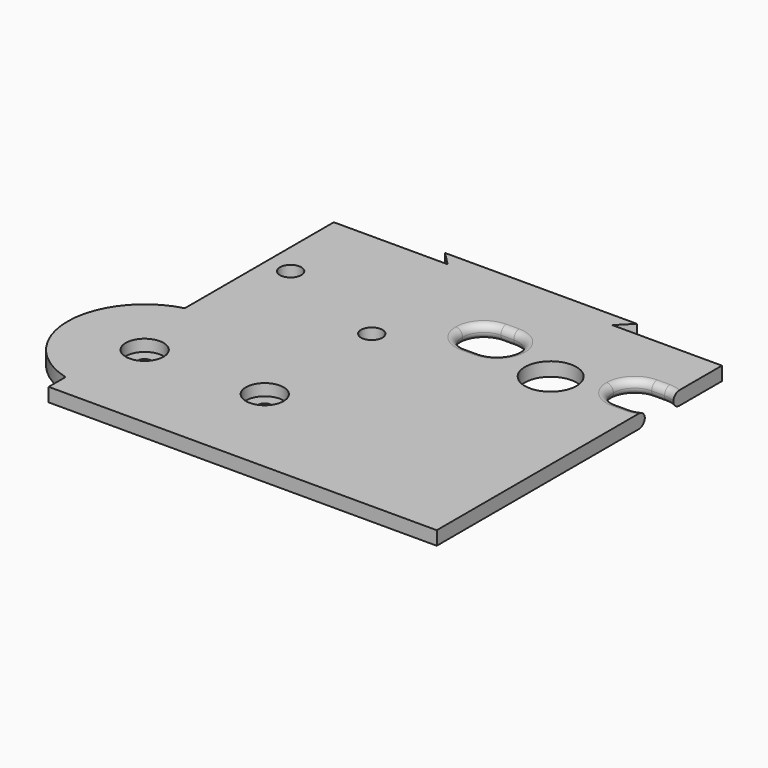
from build123d import *

# Parameters (mm, degrees)
F0_W     = 71.9074
F0_H     = 33.4264
F0_R     = 1.9812
F0_R_2   = 4.7752
F0_R_3   = 1.27
F1_DEPTH = 2.54
F3_DEPTH = 25.4
F4_W     = 35.56
F4_H     = 2.54
F5_DEPTH = 2.54
F7_DEPTH = 2.54
F8_R     = 3.4925
F8_R_2   = 1.27
F9_DEPTH = 2.159
F10_R    = 1.26999


# Not quite as in the source:
# - a fillet or chamfer is up to 0.001 mm smaller than in the source, because OpenCascade refuses the exact size


with BuildPart() as f1:
    # F0 (on Top) → F1 (new body)
    with BuildSketch(Plane.XY):
        with Locations((35.9537, 16.7132)):
            Rectangle(F0_W, F0_H)
        with Locations((26.1112, 9.5758)):
            Circle(F0_R, mode=Mode.SUBTRACT)
        with Locations((4.699, 17.5514)):
            Circle(F0_R, mode=Mode.SUBTRACT)
        with Locations((54.6862, 15.2908)):
            Circle(F0_R_2, mode=Mode.SUBTRACT)
        Polygon((71.9074, 0), (0, 0), (0, -1.0727777636), (0, -28.6960222364), (0, -32.6136), (71.9074, -32.6136), align=None)
        with Locations((3.6068, -14.8844)):
            Circle(F0_R_3, mode=Mode.SUBTRACT)
        with Locations((25.8572, -14.8844)):
            Circle(F0_R_3, mode=Mode.SUBTRACT)
        with BuildLine():
            Line((0, -28.6960222364), (0, -1.0727777636))
            ThreePointArc((0, -1.0727777636), (-10.668, -14.8844), (0, -28.6960222364))
        make_face()
    extrude(amount=F1_DEPTH)

    # F2 (on face) → F3 (cut)
    with BuildSketch(Plane.XY):
        with BuildLine():
            ThreePointArc((73.7104990378, 18.8731995366), (72.5573784353, 21.6570789342), (69.7734990378, 22.8101995366))
            Line((69.7734990378, 22.8101995366), (67.3858990378, 22.8101995366))
            ThreePointArc((67.3858990378, 22.8101995366), (64.6020196402, 21.6570789342), (63.4488990378, 18.8731995366))
            ThreePointArc((63.4488990378, 18.8731995366), (64.6020196402, 16.0893201391), (67.3858990378, 14.9361995366))
            Line((67.3858990378, 14.9361995366), (69.7734990378, 14.9361995366))
            ThreePointArc((69.7734990378, 14.9361995366), (72.5573784353, 16.0893201391), (73.7104990378, 18.8731995366))
        make_face()
        with BuildLine():
            ThreePointArc((45.7704990378, 18.8731995366), (44.6173784353, 21.6570789342), (41.8334990378, 22.8101995366))
            Line((41.8334990378, 22.8101995366), (39.4458990378, 22.8101995366))
            ThreePointArc((39.4458990378, 22.8101995366), (36.6620196402, 21.6570789342), (35.5088990378, 18.8731995366))
            ThreePointArc((35.5088990378, 18.8731995366), (36.6620196402, 16.0893201391), (39.4458990378, 14.9361995366))
            Line((39.4458990378, 14.9361995366), (41.8334990378, 14.9361995366))
            ThreePointArc((41.8334990378, 14.9361995366), (44.6173784353, 16.0893201391), (45.7704990378, 18.8731995366))
        make_face()
    extrude(amount=F3_DEPTH, mode=Mode.SUBTRACT)

    # F4 (on face) → F5 (join)
    with BuildSketch(Plane(origin=(0, 33.4264, 0), x_dir=(-1, 0, 0), z_dir=(0, 1, 0))):
        with Locations((-36.3474, 1.27)):
            Rectangle(F4_W, F4_H)
    extrude(amount=F5_DEPTH)

    # F6 (on face) → F7 (cut)
    with BuildSketch(Plane.XY.offset(2.54)):
        Polygon((18.5674, 33.4264), (21.1074, 33.4264), (18.5674, 35.9664), align=None)
        Polygon((54.1274, 33.4264), (54.1274, 35.9664), (51.5874, 33.4264), align=None)
    extrude(amount=-F7_DEPTH, mode=Mode.SUBTRACT)

    # F8 (on face) → F9 (cut)
    with BuildSketch(Plane.XY.offset(2.54)):
        with Locations((3.6068, -14.8844)):
            Circle(F8_R)
        with Locations((3.6068, -14.8844)):
            Circle(F8_R_2, mode=Mode.SUBTRACT)
        with Locations((25.8572, -14.8844)):
            Circle(F8_R)
        with Locations((25.8572, -14.8844)):
            Circle(F8_R_2, mode=Mode.SUBTRACT)
    extrude(amount=-F9_DEPTH, mode=Mode.SUBTRACT)

    # F10 (radius 1.27 in the source; OpenCascade refuses exactly that, so slightly less here)
    f10_edges = [f1.edges().sort_by_distance(p)[0] for p in [
        (35.508899, 18.8732, 2.54),
        (63.448899, 18.8732, 2.54),
        (63.448899, 18.8732, 0),
        (45.770499, 18.8732, 0),
    ]]
    fillet(f10_edges, radius=F10_R)


solid = f1.part
